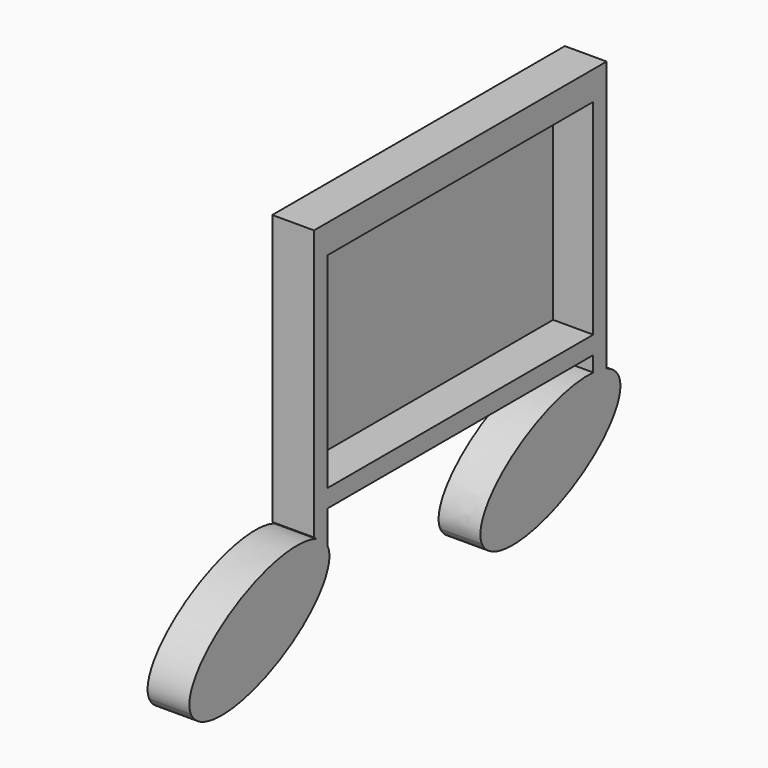
from build123d import *

# Parameters (mm, degrees)
F1_DEPTH = 25
F0_W     = 10
F0_H     = 10.7577247995
F0_H_2   = 122.6931678566
F0_H_3   = 17.192529671
F2_DEPTH = 25
F4_W     = 198.9417937062
F4_H     = 122.6931678566
F5_DEPTH = 1


with BuildPart() as f1:
    # F0 (on Right) → F1 (new body)
    with BuildSketch(Plane.YZ):
        with BuildLine():
            add(Edge.make_bspline(
                [(-24.8732831738, -8.3684676666), (-27.2337296254, -4.0002896584), (-32.9585265225, -1.6023579126)],
                knots=[3.1735872833, 3.1735872833, 3.1735872833, 3.5481673673, 3.5481673673, 3.5481673673], degree=2, weights=[1, 0.9825124283, 1]))
            Line((-32.9585265225, -1.6023579126), (-24.8732831738, -8.3684676666))
        make_face()
        with BuildLine():
            Line((-24.8732831738, -8.3684676666), (-32.9585265225, -1.6023579126))
            add(Edge.make_bspline(
                [(-32.9585265225, -1.6023579126), (-57.5749186792, 8.7086503695), (-96.7004471766, -13.8016316094), (-135.825975674, -36.3119135884), (-127.0076956824, -55.7121271344)],
                knots=[3.5481673673, 3.5481673673, 3.5481673673, 4.9156763373, 4.9156763373, 6.2831853072, 6.2831853072, 6.2831853072], degree=2, weights=[1, 0.77520645, 1, 0.77520645, 1]))
            add(Edge.make_bspline(
                [(-127.0076956824, -55.7121271344), (-116.0117459205, -79.9032135735), (-64.1143561941, -55.8465583666), (-12.2169664676, -31.7899031597), (-24.8732831738, -8.3684676666)],
                knots=[0, 0, 0, 1.5867936416, 1.5867936416, 3.1735872833, 3.1735872833, 3.1735872833], degree=2, weights=[1, 0.7014283169, 1, 0.7014283169, 1]))
        make_face()
    extrude(amount=F1_DEPTH)

    # F0 (on Right) → F2 (join)
    with BuildSketch(Plane.YZ):
        with BuildLine():
            Line((-34.8732831738, 11.1536691385), (-34.8732831738, 0))
            Line((-34.8732831738, 0), (-32.9585265225, -1.6023579126))
            add(Edge.make_bspline(
                [(-24.8732831738, -8.3684676666), (-27.2337296254, -4.0002896584), (-32.9585265225, -1.6023579126)],
                knots=[3.1735872833, 3.1735872833, 3.1735872833, 3.5481673673, 3.5481673673, 3.5481673673], degree=2, weights=[1, 0.9825124283, 1]))
            Line((-24.8732831738, -8.3684676666), (-24.8732831738, 11.1536691385))
            Line((-24.8732831738, 11.1536691385), (-34.8732831738, 11.1536691385))
        make_face()
        with Locations((-29.8732831738, 16.5325315383)):
            Rectangle(F0_W, F0_H)
        with BuildLine():
            Line((-24.8732831738, -8.3684676666), (-32.9585265225, -1.6023579126))
            add(Edge.make_bspline(
                [(-32.9585265225, -1.6023579126), (-57.5749186792, 8.7086503695), (-96.7004471766, -13.8016316094), (-135.825975674, -36.3119135884), (-127.0076956824, -55.7121271344)],
                knots=[3.5481673673, 3.5481673673, 3.5481673673, 4.9156763373, 4.9156763373, 6.2831853072, 6.2831853072, 6.2831853072], degree=2, weights=[1, 0.77520645, 1, 0.77520645, 1]))
            add(Edge.make_bspline(
                [(-127.0076956824, -55.7121271344), (-116.0117459205, -79.9032135735), (-64.1143561941, -55.8465583666), (-12.2169664676, -31.7899031597), (-24.8732831738, -8.3684676666)],
                knots=[0, 0, 0, 1.5867936416, 1.5867936416, 3.1735872833, 3.1735872833, 3.1735872833], degree=2, weights=[1, 0.7014283169, 1, 0.7014283169, 1]))
        make_face()
        with BuildLine():
            add(Edge.make_bspline(
                [(-24.8732831738, -8.3684676666), (-27.2337296254, -4.0002896584), (-32.9585265225, -1.6023579126)],
                knots=[3.1735872833, 3.1735872833, 3.1735872833, 3.5481673673, 3.5481673673, 3.5481673673], degree=2, weights=[1, 0.9825124283, 1]))
            Line((-32.9585265225, -1.6023579126), (-24.8732831738, -8.3684676666))
        make_face()
        with Locations((-29.8732831738, 83.2579778663)):
            Rectangle(F0_W, F0_H_2)
        Polygon((-24.8732831738, 21.911393938), (-24.8732831738, 11.1536691385), (174.0685105324, 11.1536691385), (174.0685105324, 21.911393938), (77.5494836288, 21.911393938), (66.2534190328, 21.911393938), align=None)
        with Locations((-29.8732831738, 153.2008266301)):
            Rectangle(F0_W, F0_H_3)
        with Locations((179.0685105324, 16.5325315383)):
            Rectangle(F0_W, F0_H)
        Polygon((184.0685105324, 11.1536691385), (174.0685105324, 11.1536691385), (174.0685105324, 5.1707883091), (184.0685105324, 0), (184.0685105324, 2.2556344343), align=None)
        Polygon((-24.8732831738, 161.7970914655), (-24.8732831738, 144.6045617946), (66.2534190328, 144.6045617946), (77.5494836288, 144.6045617946), (174.0685105324, 144.6045617946), (174.0685105324, 161.7970914655), align=None)
        with Locations((179.0685105324, 83.2579778663)):
            Rectangle(F0_W, F0_H_2)
        with BuildLine():
            Line((184.0685105324, 0), (174.0685105324, 5.1707883091))
            Line((174.0685105324, 5.1707883091), (174.0685105324, 1.9807628364))
            add(Edge.make_bspline(
                [(183.5856257709, 0.095648019), (179.4483388614, 1.5818426104), (174.0685105324, 1.9807628364)],
                knots=[3.5871608427, 3.5871608427, 3.5871608427, 3.8454834836, 3.8454834836, 3.8454834836], degree=2, weights=[1, 0.9916702665, 1]))
            Line((183.5856257709, 0.095648019), (184.0685105324, 0))
        make_face()
        with Locations((179.0685105324, 153.2008266301)):
            Rectangle(F0_W, F0_H_3)
        with BuildLine():
            Line((183.5856257709, 0.095648019), (174.0685105324, 1.9807628364))
            add(Edge.make_bspline(
                [(174.0685105324, 1.9807628364), (61.2792557287, 10.3442109358), (90.7466135574, -54.4839681489)],
                knots=[3.8454834836, 3.8454834836, 3.8454834836, 6.2831853072, 6.2831853072, 6.2831853072], degree=2, weights=[1, 0.3447246272, 1]))
            add(Edge.make_bspline(
                [(90.7466135574, -54.4839681489), (104.2938042759, -84.2877839883), (163.8782388313, -49.2583767372), (223.4626733866, -14.2289694862), (183.5856257709, 0.095648019)],
                knots=[0, 0, 0, 1.7935804213, 1.7935804213, 3.5871608427, 3.5871608427, 3.5871608427], degree=2, weights=[1, 0.6241210762, 1, 0.6241210762, 1]))
        make_face()
        with BuildLine():
            add(Edge.make_bspline(
                [(183.5856257709, 0.095648019), (179.4483388614, 1.5818426104), (174.0685105324, 1.9807628364)],
                knots=[3.5871608427, 3.5871608427, 3.5871608427, 3.8454834836, 3.8454834836, 3.8454834836], degree=2, weights=[1, 0.9916702665, 1]))
            Line((174.0685105324, 1.9807628364), (183.5856257709, 0.095648019))
        make_face()
    extrude(amount=F2_DEPTH)

    # F4 (on offset) → F5 (join)
    with BuildSketch(Plane(origin=(0, 0, 0), x_dir=(0, -1, 0), z_dir=(-1, 0, 0))):
        with Locations((-74.5976136793, 83.2579778663)):
            Rectangle(F4_W, F4_H)
    extrude(amount=-F5_DEPTH)


solid = f1.part
